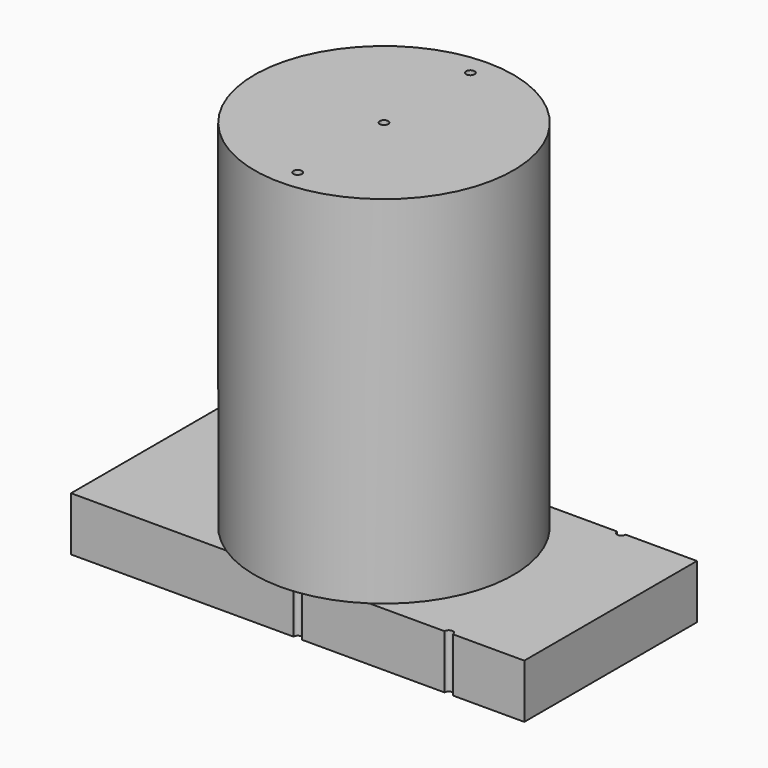
from build123d import *

# Parameters (mm, degrees)
F0_W     = 266.7
F0_H     = 127
F1_DEPTH = 31.75
F3_DEPTH = 209.55
F4_D     = 5


with BuildPart() as f1:
    # F0 (on Top) → F1 (new body)
    with BuildSketch(Plane.XY):
        Rectangle(F0_W, F0_H)
    extrude(amount=F1_DEPTH)

    # F2 (on face) → F3 (join)
    with BuildSketch(Plane.XY.offset(31.75)):
        with BuildLine():
            Line((-42.1211348375, 63.5), (42.1211348375, 63.5))
            ThreePointArc((42.1211348375, 63.5), (0, 76.2), (-42.1211348375, 63.5))
        make_face()
        with BuildLine():
            ThreePointArc((42.1211348375, -63.5), (67.1419037361, -36.0333840028), (76.2, 0))
            ThreePointArc((76.2, 0), (67.1419037361, 36.0333840028), (42.1211348375, 63.5))
            Line((42.1211348375, 63.5), (-42.1211348375, 63.5))
            ThreePointArc((-42.1211348375, 63.5), (-76.2, 0), (-42.1211348375, -63.5))
            Line((-42.1211348375, -63.5), (42.1211348375, -63.5))
        make_face()
        with BuildLine():
            ThreePointArc((-42.1211348375, -63.5), (0, -76.2), (42.1211348375, -63.5))
            Line((42.1211348375, -63.5), (-42.1211348375, -63.5))
        make_face()
    extrude(amount=F3_DEPTH)

    # F4 (through all)
    with Locations(Plane(origin=(0, 0, 0), x_dir=(1, 0, 0), z_dir=(0, 0, -1))):
        with Locations((88.9, -63.5), (88.9, 63.5), (0, 63.5), (0, -63.5), (0, 0)):
            Hole(F4_D / 2)


solid = f1.part
